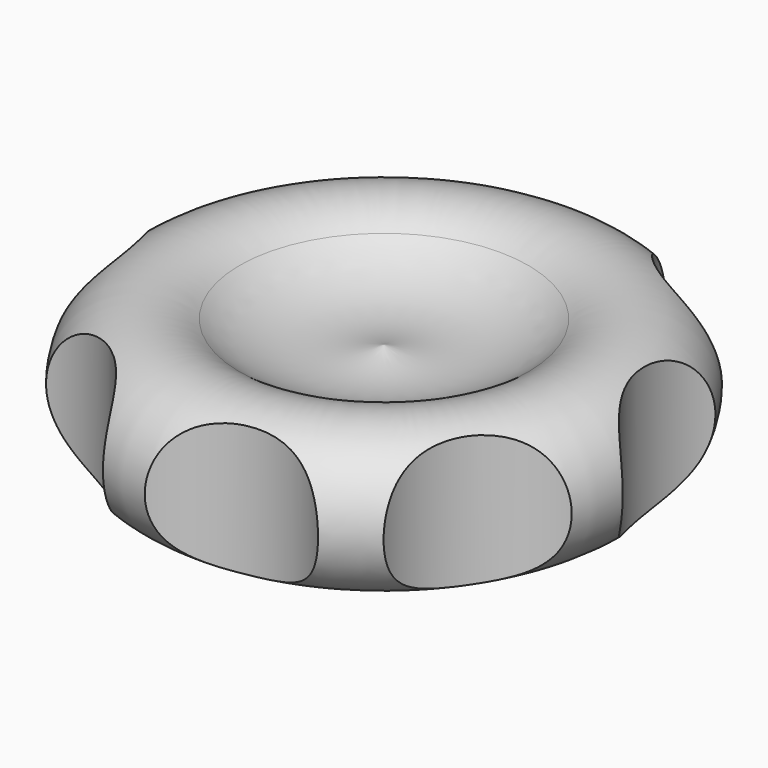
from build123d import *
from build123d import SkipClean  # not in build123d's __all__

# Parameters (mm, degrees)
F2_R     = 16.1667504952
F3_DEPTH = 41.656


with BuildPart() as f1:
    # F0 (on Front) → F1 (revolve)
    with BuildSketch(Plane.XZ):
        with BuildLine():
            ThreePointArc((0, 14.9591247887), (-10.3684434411, 13.8941619175), (-19.9058614508, 18.0984957548))
            ThreePointArc((-19.9058614508, 18.0984957548), (-35.8352260418, 13.5193513609), (-26.2466725307, 0))
            Line((-26.2466725307, 0), (0, 0))
            Line((0, 0), (0, 14.9591247887))
        make_face()
    revolve(axis=Axis((0, 0, 7.4990492945), (0, 0, -1)))

    # F2 (on Top) → F3 (cut)
    with BuildSketch(Plane.XY):
        with Locations((-8.5725001991, 46.2642833591)):
            Circle(F2_R)
        with Locations((-38.7754615124, 26.6521154674)):
            Circle(F2_R)
        with Locations((-46.2642833591, -8.5725001991)):
            Circle(F2_R)
        with Locations((-26.6521154674, -38.7754615124)):
            Circle(F2_R)
        with Locations((8.5725001991, -46.2642833591)):
            Circle(F2_R)
        with Locations((38.7754615124, -26.6521154674)):
            Circle(F2_R)
        with Locations((46.2642833591, 8.5725001991)):
            Circle(F2_R)
        with Locations((26.6521154674, 38.7754615124)):
            Circle(F2_R)
    with SkipClean():  # cleaning this boolean's faces spoils the solid; the shape is the same uncleaned
        extrude(amount=F3_DEPTH, mode=Mode.SUBTRACT)


solid = f1.part
